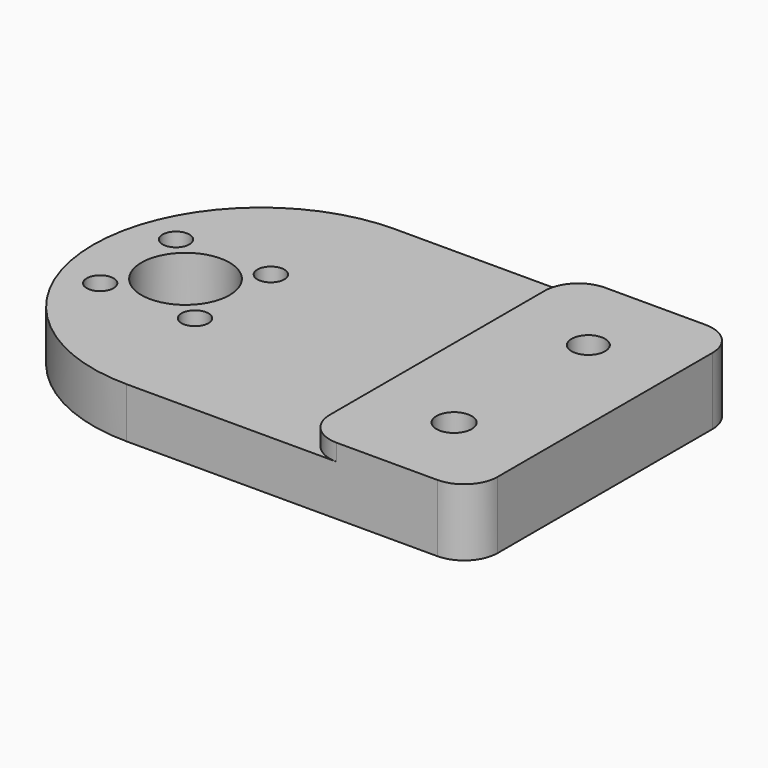
from build123d import *

# Parameters (mm, degrees)
F0_W     = 61
F0_H     = 40
F0_R     = 1.6
F0_R_2   = 2.1
F0_R_3   = 5.25
F0_R_4   = 2
F1_DEPTH = 6
F2_DEPTH = 77
F3_R     = 19.99999
F4_W     = 20
F4_H     = 40
F4_R     = 2.1
F4_R_2   = 2
F5_DEPTH = 2
F6_R     = 4


# Not quite as in the source:
# - a fillet or chamfer is up to 0.001 mm smaller than in the source, because OpenCascade refuses the exact size
# - an extrude ends at something that could not be found from the text; its depth is read off the source's solid


with BuildPart() as f1:
    # F0 (on Top) → F1 (new body)
    with BuildSketch(Plane.XY):
        Rectangle(F0_W, F0_H)
        with Locations((-25.15, -5.65)):
            Circle(F0_R, mode=Mode.SUBTRACT)
        with Locations((-13.85, -5.65)):
            Circle(F0_R, mode=Mode.SUBTRACT)
        with Locations((20.5, -10)):
            Circle(F0_R_2, mode=Mode.SUBTRACT)
        with Locations((-19.5, 0)):
            Circle(F0_R_3, mode=Mode.SUBTRACT)
        with Locations((-25.15, 5.65)):
            Circle(F0_R, mode=Mode.SUBTRACT)
        with Locations((-13.85, 5.65)):
            Circle(F0_R, mode=Mode.SUBTRACT)
        with Locations((20.5, 10)):
            Circle(F0_R_4, mode=Mode.SUBTRACT)
    extrude(amount=F1_DEPTH)

    # F0 (on Top) → F2 (cut, through all)
    with BuildSketch(Plane.XY):
        Rectangle(F0_W, F0_H)
        with Locations((-25.15, -5.65)):
            Circle(F0_R, mode=Mode.SUBTRACT)
        with Locations((-13.85, -5.65)):
            Circle(F0_R, mode=Mode.SUBTRACT)
        with Locations((20.5, -10)):
            Circle(F0_R_2, mode=Mode.SUBTRACT)
        with Locations((-19.5, 0)):
            Circle(F0_R_3, mode=Mode.SUBTRACT)
        with Locations((-25.15, 5.65)):
            Circle(F0_R, mode=Mode.SUBTRACT)
        with Locations((-13.85, 5.65)):
            Circle(F0_R, mode=Mode.SUBTRACT)
        with Locations((20.5, 10)):
            Circle(F0_R_4, mode=Mode.SUBTRACT)
    extrude(amount=-F2_DEPTH, mode=Mode.SUBTRACT)

    # F3 (radius 20 in the source; OpenCascade refuses exactly that, so slightly less here)
    f3_edges = [f1.edges().sort_by_distance(p)[0] for p in [
        (-30.5, -20, 3),
        (-30.5, 20, 3),
    ]]
    fillet(f3_edges, radius=F3_R)

    # F4 (on face) → F5 (join)
    with BuildSketch(Plane.XY.offset(6)):
        with Locations((20.5, 0)):
            Rectangle(F4_W, F4_H)
        with Locations((20.5, -10)):
            Circle(F4_R, mode=Mode.SUBTRACT)
        with Locations((20.5, 10)):
            Circle(F4_R_2, mode=Mode.SUBTRACT)
    extrude(amount=F5_DEPTH)

    # F6
    f6_edges = [f1.edges().sort_by_distance(p)[0] for p in [
        (10.5, -20, 7),
        (30.5, -20, 4),
        (10.5, 20, 7),
        (30.5, 20, 4),
    ]]
    fillet(f6_edges, radius=F6_R)


solid = f1.part
